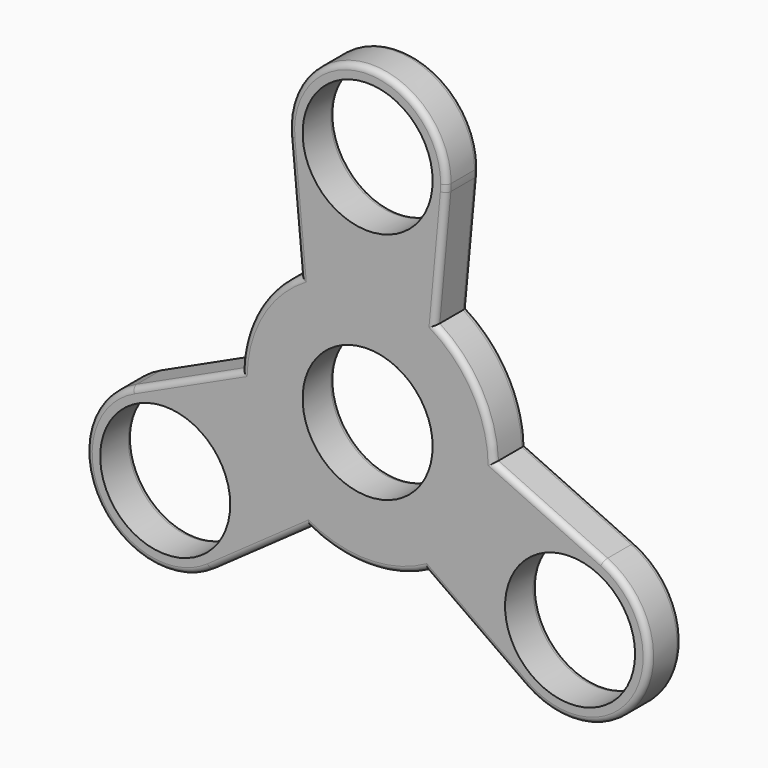
from build123d import *

# Parameters (mm, degrees)
F0_R     = 11.125
F1_DEPTH = 7
F2_R     = 1


# Not quite as in the source:
# - a feature names something its author has since deleted; it is built from what else it names


with BuildPart() as f1:
    # F0 (on Front) → F1 (new body)
    with BuildSketch(Plane.XZ):
        with BuildLine():
            ThreePointArc((0, 16.5), (6.7082039325, 14.2177978871), (10.632866558, 8.3181818182))
            Line((10.632866558, 8.3181818182), (11.5520522489, 18.27584709))
            Line((11.5520522489, 18.27584709), (13.442848117, 38.7590993172))
            ThreePointArc((13.442848117, 38.7590993172), (0, 26.5), (-13.442848117, 38.7590993172))
            Line((-13.442848117, 38.7590993172), (-11.5520522489, 18.27584709))
            Line((-11.5520522489, 18.27584709), (-10.632866558, 8.3181818182))
            ThreePointArc((-10.632866558, 8.3181818182), (-6.7082039325, 14.2177978871), (0, 16.5))
        make_face()
        with BuildLine():
            ThreePointArc((-1.8873234889, -13.3674234633), (-14.2894191624, -8.25), (-12.5201900468, 5.0492416452))
            Line((-12.5201900468, 5.0492416452), (-21.6033739801, 0.8664471684))
            Line((-21.6033739801, 0.8664471684), (-40.287788695, -7.7377016901))
            ThreePointArc((-40.287788695, -7.7377016901), (-27.3602685709, -8.6315913748), (-21.1410161514, -20))
            ThreePointArc((-21.1410161514, -20), (-22.6514994755, -26.2049568798), (-26.844940578, -31.0213976271))
            Line((-26.844940578, -31.0213976271), (-10.0513217312, -19.1422942584))
            Line((-10.0513217312, -19.1422942584), (-1.8873234889, -13.3674234633))
        make_face()
        with BuildLine():
            ThreePointArc((1.8873234889, -13.3674234633), (14.2894191624, -8.25), (12.5201900468, 5.0492416452))
            ThreePointArc((12.5201900468, 5.0492416452), (13.2527839647, 2.5717148333), (13.5, 0))
            ThreePointArc((13.5, 0), (10.1913901677, -8.8535623593), (1.8873234889, -13.3674234633))
        make_face()
        with BuildLine():
            ThreePointArc((-1.8873234889, -13.3674234633), (-11.6913429511, -6.75), (-12.5201900468, 5.0492416452))
            ThreePointArc((-12.5201900468, 5.0492416452), (-14.2894191624, -8.25), (-1.8873234889, -13.3674234633))
        make_face()
        with BuildLine():
            Line((0, 16.5), (0, 13.5))
            ThreePointArc((0, 13.5), (5.9141586661, 12.1355975243), (10.632866558, 8.3181818182))
            ThreePointArc((10.632866558, 8.3181818182), (6.7082039325, 14.2177978871), (0, 16.5))
        make_face()
        with BuildLine():
            Line((21.6033739801, 0.8664471684), (12.5201900468, 5.0492416452))
            ThreePointArc((12.5201900468, 5.0492416452), (14.2894191624, -8.25), (1.8873234889, -13.3674234633))
            Line((1.8873234889, -13.3674234633), (10.0513217312, -19.1422942584))
            Line((10.0513217312, -19.1422942584), (26.844940578, -31.0213976271))
            ThreePointArc((26.844940578, -31.0213976271), (22.9496732003, -13.25), (40.287788695, -7.7377016901))
            Line((40.287788695, -7.7377016901), (21.6033739801, 0.8664471684))
        make_face()
        with BuildLine():
            ThreePointArc((-10.632866558, 8.3181818182), (-5.9141586661, 12.1355975243), (0, 13.5))
            Line((0, 13.5), (0, 16.5))
            ThreePointArc((0, 16.5), (-6.7082039325, 14.2177978871), (-10.632866558, 8.3181818182))
        make_face()
        with BuildLine():
            ThreePointArc((-13.442848117, 38.7590993172), (0, 26.5), (13.442848117, 38.7590993172))
            ThreePointArc((13.442848117, 38.7590993172), (13.4857044603, 39.3788919494), (13.5, 40))
            ThreePointArc((13.5, 40), (-0.6211080506, 53.4857044603), (-13.442848117, 38.7590993172))
        make_face()
        with Locations((0, 40)):
            Circle(F0_R, mode=Mode.SUBTRACT)
        with BuildLine():
            ThreePointArc((10.632866558, 8.3181818182), (5.9141586661, 12.1355975243), (0, 13.5))
            ThreePointArc((0, 13.5), (-5.9141586661, 12.1355975243), (-10.632866558, 8.3181818182))
            ThreePointArc((-10.632866558, 8.3181818182), (-11.6913429511, 6.75), (-12.5201900468, 5.0492416452))
            ThreePointArc((-12.5201900468, 5.0492416452), (-11.6913429511, -6.75), (-1.8873234889, -13.3674234633))
            ThreePointArc((-1.8873234889, -13.3674234633), (0, -13.5), (1.8873234889, -13.3674234633))
            ThreePointArc((1.8873234889, -13.3674234633), (10.1913901677, -8.8535623593), (13.5, 0))
            ThreePointArc((13.5, 0), (13.2527839647, 2.5717148333), (12.5201900468, 5.0492416452))
            ThreePointArc((12.5201900468, 5.0492416452), (11.6913429511, 6.75), (10.632866558, 8.3181818182))
        make_face()
        with BuildLine():
            ThreePointArc((0, 11.125), (7.8665629407, 7.8665629407), (11.125, 0))
            ThreePointArc((11.125, 0), (-7.8665629407, -7.8665629407), (0, 11.125))
        make_face(mode=Mode.SUBTRACT)
        with BuildLine():
            ThreePointArc((-21.1410161514, -20), (-27.3602685709, -8.6315913748), (-40.287788695, -7.7377016901))
            ThreePointArc((-40.287788695, -7.7377016901), (-46.3323591025, -26.75), (-26.844940578, -31.0213976271))
            ThreePointArc((-26.844940578, -31.0213976271), (-22.6514994755, -26.2049568798), (-21.1410161514, -20))
        make_face()
        with Locations((-34.6410161514, -20)):
            Circle(F0_R, mode=Mode.SUBTRACT)
        with BuildLine():
            ThreePointArc((48.1410161514, -20), (46.0094247766, -12.7192524195), (40.287788695, -7.7377016901))
            ThreePointArc((40.287788695, -7.7377016901), (22.9496732003, -13.25), (26.844940578, -31.0213976271))
            ThreePointArc((26.844940578, -31.0213976271), (40.8459730312, -31.9895166758), (48.1410161514, -20))
        make_face()
        with Locations((34.6410161514, -20)):
            Circle(F0_R, mode=Mode.SUBTRACT)
        with BuildLine():
            ThreePointArc((-12.5201900468, 5.0492416452), (-11.6913429511, 6.75), (-10.632866558, 8.3181818182))
            Line((-10.632866558, 8.3181818182), (-11.5520522489, 18.27584709))
            ThreePointArc((-11.5520522489, 18.27584709), (-18.7241120888, 10.8103711548), (-21.6033739801, 0.8664471684))
            Line((-21.6033739801, 0.8664471684), (-12.5201900468, 5.0492416452))
        make_face()
        with BuildLine():
            Line((11.5520522489, 18.27584709), (10.632866558, 8.3181818182))
            ThreePointArc((10.632866558, 8.3181818182), (11.6913429511, 6.75), (12.5201900468, 5.0492416452))
            Line((12.5201900468, 5.0492416452), (21.6033739801, 0.8664471684))
            ThreePointArc((21.6033739801, 0.8664471684), (18.7241120888, 10.8103711548), (11.5520522489, 18.27584709))
        make_face()
        with BuildLine():
            Line((10.0513217312, -19.1422942584), (1.8873234889, -13.3674234633))
            ThreePointArc((1.8873234889, -13.3674234633), (0, -13.5), (-1.8873234889, -13.3674234633))
            Line((-1.8873234889, -13.3674234633), (-10.0513217312, -19.1422942584))
            ThreePointArc((-10.0513217312, -19.1422942584), (0, -21.6207423096), (10.0513217312, -19.1422942584))
        make_face()
    extrude(amount=F1_DEPTH)

    # F2
    f2_edges = [f1.edges().sort_by_distance(p)[0] for p in [
        (12.49745, -7, 28.517473),
        (-30.945581, -7, -3.435627),
        (18.448131, -7, -25.081846),
        (-18.448131, 0, -25.081846),
        (-12.49745, 0, 28.517473),
        (-18.724112, 0, 10.810371),
        (-30.945581, 0, -3.435627),
        (-46.332359, 0, -26.75),
        (0, 0, -21.620742),
        (18.448131, 0, -25.081846),
        (46.332359, 0, -26.75),
        (30.945581, 0, -3.435627),
        (18.724112, 0, 10.810371),
        (12.49745, 0, 28.517473),
        (0, 0, 53.5),
        (-11.125, 0, 40),
        (-11.125, 0, 0),
        (-45.766016, 0, -20),
        (23.516016, 0, -20),
        (18.724112, -7, 10.810371),
        (0, -7, -21.620742),
        (-18.724112, -7, 10.810371),
    ]]
    fillet(f2_edges, radius=F2_R)


solid = f1.part
